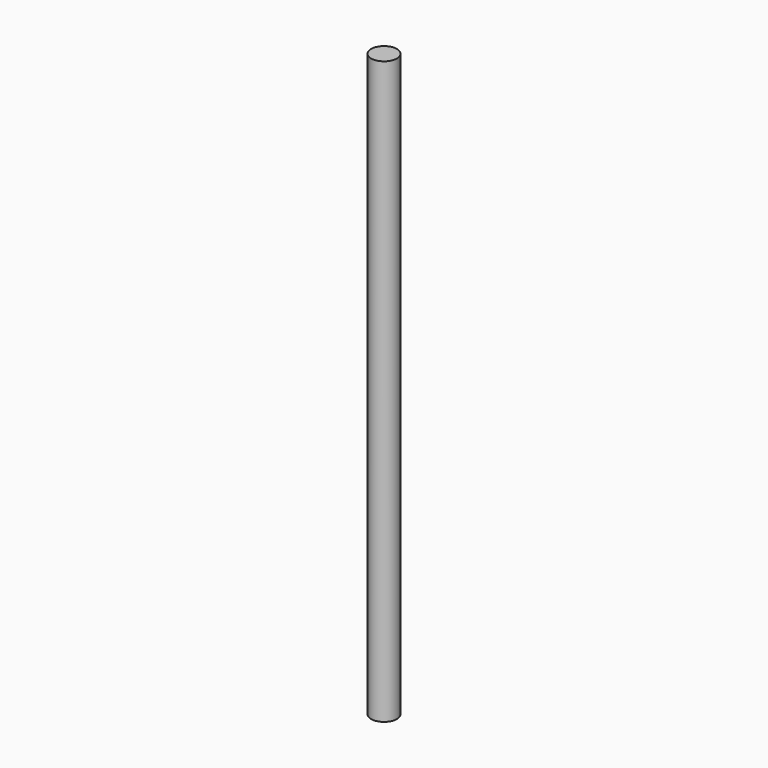
from build123d import *

# Parameters (mm, degrees)
F0_R     = 12.7
F2_DEPTH = 571.5


# Not quite as in the source:
# - the program builds the solid bodies; features that only make, move or delete a surface that nothing else refers to are left out


with BuildPart() as f2:
    # F0 (on Top) → F2 (new body)
    with BuildSketch(Plane.XY):
        Circle(F0_R)
    extrude(amount=-F2_DEPTH)


solid = f2.part
